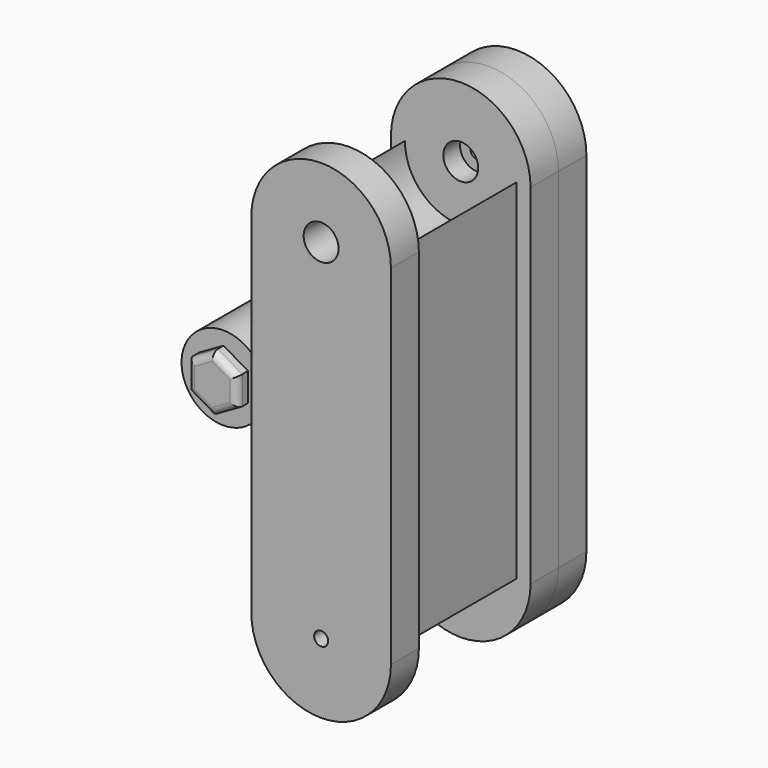
from build123d import *
from build123d import SkipClean  # not in build123d's __all__

# Parameters (mm, degrees)
F0_W      = 20
F0_H      = 25
F1_DEPTH  = 16
F3_DEPTH  = 20.001
F5_DEPTH  = 5
F6_R      = 2.5
F7_DEPTH  = 3
F8_R      = 1
F9_DEPTH  = 2.001
F11_R     = 2.5
F12_DEPTH = 5
F13_R     = 2.5
F14_DEPTH = 3
F15_R     = 1
F16_DEPTH = 2.001
F18_DEPTH = 5
F19_R     = 2.5
F20_DEPTH = 25.001
F21_R     = 2.5
F22_DEPTH = 3
F23_R     = 1
F25_DEPTH = 5
F26_R     = 6
F27_DEPTH = 20
F28_R     = 2.5
F29_DEPTH = 40.4173054965
F31_DEPTH = 2
F32_R     = 1
F33_R     = 2.25
F34_DEPTH = 25
F35_W     = 2
F35_H     = 20
F36_DEPTH = 15
F37_R     = 5
F38_R     = 2.25
F39_DEPTH = 7.0441698188


with BuildPart() as f1:
    # F0 (on Right) → F1 (new body)
    with BuildSketch(Plane.YZ):
        with Locations((0, -12.5)):
            Rectangle(F0_W, F0_H)
    extrude(amount=F1_DEPTH)

    # F2 (on face) → F3 (cut, through all)
    with BuildSketch(Plane(origin=(0, 10, 0), x_dir=(-1, 0, 0), z_dir=(0, 1, 0))):
        with BuildLine():
            Line((-16, -25), (0, -25))
            ThreePointArc((0, -25), (-8, -17), (-16, -25))
        make_face()
    extrude(amount=-F3_DEPTH, mode=Mode.SUBTRACT)

    # F4 (on face) → F5 (join)
    with BuildSketch(Plane(origin=(0, 10, 0), x_dir=(-1, 0, 0), z_dir=(0, 1, 0))):
        with BuildLine():
            Line((-18, 0), (-18, -25))
            ThreePointArc((-18, -25), (-8, -35), (2, -25))
            Line((2, -25), (2, 0))
            Line((2, 0), (-18, 0))
        make_face()
    extrude(amount=F5_DEPTH)

    # F6 (on face) → F7 (cut)
    with BuildSketch(Plane.XZ.offset(-10)):
        with Locations((8, -25)):
            Circle(F6_R)
    extrude(amount=-F7_DEPTH, mode=Mode.SUBTRACT)

    # F8 (on face) → F9 (cut, through all)
    with BuildSketch(Plane.XZ.offset(-13)):
        with Locations((8, -25)):
            Circle(F8_R)
    extrude(amount=-F9_DEPTH, mode=Mode.SUBTRACT)

    # F10: F1 across plane


with BuildPart() as f1_1:
    add(f1.part, clean=False)
    add(f1.part.mirror(Plane.XY), clean=False)

    # F17 (on face) → F18 (join)
    with BuildSketch(Plane(origin=(-2, 0, 0), x_dir=(0, -1, 0), z_dir=(-1, 0, 0))):
        with BuildLine():
            Line((-28.4163054965, -8), (-20.862338065, -8))
            ThreePointArc((-20.862338065, -8), (-20.2405691294, -8.0991045819), (-19.6804203442, -8.3865966093))
            Line((-19.6804203442, -8.3865966093), (-10, -15.4781029345))
            Line((-10, -15.4781029345), (-10, -8))
            Line((-10, -8), (-10, 8))
            Line((-10, 8), (-10, 15.4781029345))
            Line((-10, 15.4781029345), (-19.6804203442, 8.3865966093))
            ThreePointArc((-19.6804203442, 8.3865966093), (-20.2405691294, 8.0991045819), (-20.862338065, 8))
            Line((-20.862338065, 8), (-28.4163054965, 8))
            ThreePointArc((-28.4163054965, 8), (-29.8305190589, 7.4142135624), (-30.4163054965, 6))
            Line((-30.4163054965, 6), (-30.4163054965, -6))
            ThreePointArc((-30.4163054965, -6), (-29.8305190589, -7.4142135624), (-28.4163054965, -8))
        make_face()
    extrude(amount=F18_DEPTH)

    # F19 (on face) → F20 (cut, through all)
    with BuildSketch(Plane(origin=(-7, 0, 0), x_dir=(0, -1, 0), z_dir=(-1, 0, 0))):
        with Locations((-25, 0)):
            Circle(F19_R)
    extrude(amount=-F20_DEPTH, mode=Mode.SUBTRACT)

    # F21 (on face) → F22 (join)
    with BuildSketch(Plane.YZ.offset(-2)):
        Polygon((26.5397279342, 3.6917797725), (22.5726888989, 3.1793333922), (21.0329609647, -0.5124463803), (23.4602720658, -3.6917797725), (27.4273111011, -3.1793333922), (28.9670390353, 0.5124463803), align=None)
        with Locations((25, 0)):
            Circle(F21_R, mode=Mode.SUBTRACT)
    with SkipClean():  # cleaning this boolean's faces spoils the solid; the shape is the same uncleaned
        extrude(amount=F22_DEPTH)

    # F23
    f23_edges = [f1_1.edges().sort_by_distance(p)[0] for p in [
        (1, 24.556208, 3.435557),
        (1, 21.802825, 1.333444),
        (1, 22.246617, -2.102113),
        (1, 25.443792, -3.435557),
        (1, 28.197175, -1.333444),
        (1, 27.753383, 2.102113),
    ]]
    fillet(f23_edges, radius=F23_R)


with BuildPart() as f12:
    # F11 (on face) → F12 (new body)
    with BuildSketch(Plane.XZ.offset(10)):
        with BuildLine():
            Line((-2, 25), (-2, -25))
            ThreePointArc((-2, -25), (8, -35), (18, -25))
            Line((18, -25), (18, 25))
            ThreePointArc((18, 25), (8, 35), (-2, 25))
        make_face()
        with BuildLine():
            Line((0, -25), (0, 25))
            ThreePointArc((0, 25), (8, 17), (16, 25))
            Line((16, 25), (16, -25))
            ThreePointArc((16, -25), (8, -17), (0, -25))
        make_face(mode=Mode.SUBTRACT)
        with Locations((8, 25)):
            Circle(F11_R, mode=Mode.SUBTRACT)
        with BuildLine():
            ThreePointArc((16, 25), (8, 17), (0, 25))
            Line((0, 25), (0, -25))
            ThreePointArc((0, -25), (8, -17), (16, -25))
            Line((16, -25), (16, 25))
        make_face()
    extrude(amount=F12_DEPTH)

    # F13 (on face) → F14 (cut)
    with BuildSketch(Plane(origin=(0, -10, 0), x_dir=(-1, 0, 0), z_dir=(0, 1, 0))):
        with Locations((-8, -25)):
            Circle(F13_R)
    extrude(amount=-F14_DEPTH, mode=Mode.SUBTRACT)

    # F15 (on face) → F16 (cut, through all)
    with BuildSketch(Plane(origin=(0, -13, 0), x_dir=(-1, 0, 0), z_dir=(0, 1, 0))):
        with Locations((-8, -25)):
            Circle(F15_R)
    extrude(amount=-F16_DEPTH, mode=Mode.SUBTRACT)


with BuildPart() as f25:
    # F24 (on face) → F25 (new body)
    with BuildSketch(Plane(origin=(0, 15, 0), x_dir=(-1, 0, 0), z_dir=(0, 1, 0))):
        with BuildLine():
            Line((-18, 25), (-18, -25))
            ThreePointArc((-18, -25), (-8, -35), (2, -25))
            Line((2, -25), (2, 25))
            ThreePointArc((2, 25), (-8, 35), (-18, 25))
        make_face()
    extrude(amount=F25_DEPTH)


with BuildPart() as f27:
    # F26 (on face) → F27 (new body)
    with BuildSketch(Plane.XZ.offset(-10)):
        with Locations((-10, 0)):
            Circle(F26_R)
    extrude(amount=F27_DEPTH)

    # F28 (on face) → F29 (cut, through all)
    with BuildSketch(Plane.XZ.offset(10)):
        with Locations((-10, 0)):
            Circle(F28_R)
    extrude(amount=-F29_DEPTH, mode=Mode.SUBTRACT)


with BuildPart() as f31:
    # F30 (on face) → F31 (new body)
    with BuildSketch(Plane.XZ.offset(10)):
        Polygon((-6.4870996044, -2.041658587), (-6.4754216, 2.0214316901), (-9.9883219956, 4.063090277), (-13.5129003956, 2.041658587), (-13.5245784, -2.0214316901), (-10.0116780044, -4.063090277), align=None)
    extrude(amount=F31_DEPTH)

    # F32
    f32_edges = [f31.edges().sort_by_distance(p)[0] for p in [
        (-11.750611, -12, 3.052374),
        (-13.518739, -12, 0.010113),
        (-11.768128, -12, -3.042261),
        (-8.249389, -12, -3.052374),
        (-6.481261, -12, -0.010113),
        (-8.231872, -12, 3.042261),
    ]]
    fillet(f32_edges, radius=F32_R)

    # F33 (on face) → F34 (join)
    with BuildSketch(Plane(origin=(0, -10, 0), x_dir=(-1, 0, 0), z_dir=(0, 1, 0))):
        with Locations((10, 0)):
            Circle(F33_R)
    extrude(amount=F34_DEPTH)

    # F35 (on face) → F36 (join)
    with BuildSketch(Plane(origin=(0, 15, 0), x_dir=(-1, 0, 0), z_dir=(0, 1, 0))):
        with Locations((9.9568301812, 0)):
            Rectangle(F35_W, F35_H)
    extrude(amount=F36_DEPTH)

    # F37
    f37_edges = [f31.edges().sort_by_distance(p)[0] for p in [
        (-9.95683, 30, 10),
        (-9.95683, 30, -10),
    ]]
    fillet(f37_edges, radius=F37_R)

    # F38 (on face) → F39 (cut, through all)
    with BuildSketch(Plane.YZ.offset(-8.9568301812)):
        with Locations((25.0207103503, 0)):
            Circle(F38_R)
    extrude(amount=-F39_DEPTH, mode=Mode.SUBTRACT)


solid = Compound([f1_1.part, f12.part, f25.part, f27.part, f31.part])
